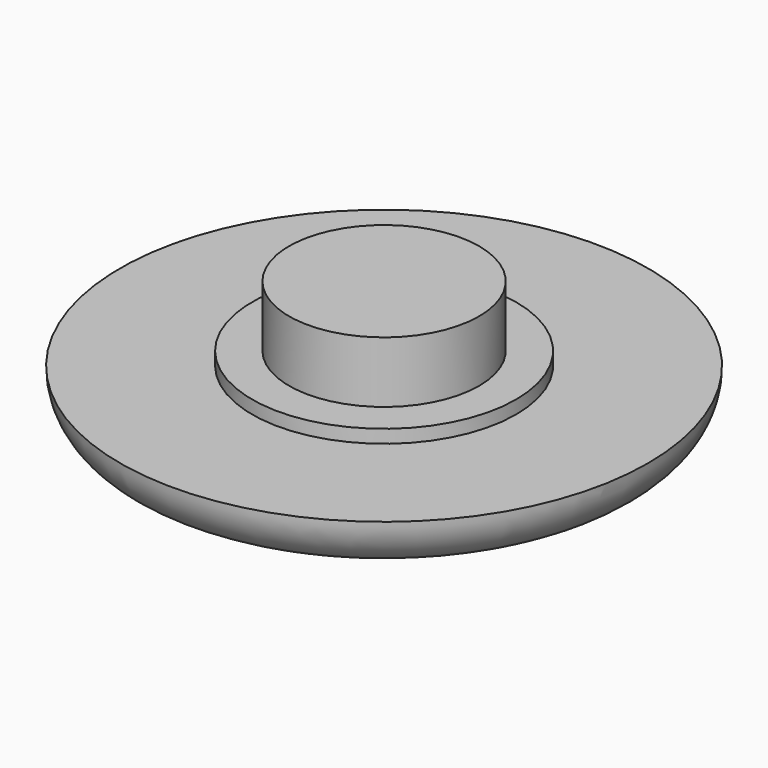
from build123d import *

# Parameters (mm, degrees)
F0_R      = 12.7
F1_DEPTH  = 2.54
F2_R      = 2.53999
F3_R      = 6.35
F4_DEPTH  = 0.635
F5_R      = 4.7625
F6_DEPTH  = 4.7244
F7_R      = 4.7625
F7_R_2    = 4.572
F8_DEPTH  = 4.7244
F9_R      = 4.572
F10_DEPTH = 1.778


# Not quite as in the source:
# - a fillet or chamfer is up to 0.001 mm smaller than in the source, because OpenCascade refuses the exact size


with BuildPart() as f1:
    # F0 (on Top) → F1 (new body)
    with BuildSketch(Plane.XY):
        Circle(F0_R)
    extrude(amount=F1_DEPTH)

    # F2 (radius 2.54 in the source; OpenCascade refuses exactly that, so slightly less here)
    f2_edges = [f1.edges().sort_by_distance(p)[0] for p in [
        (-12.7, 0, 0),
    ]]
    fillet(f2_edges, radius=F2_R)

    # F3 (on face) → F4 (join)
    with BuildSketch(Plane.XY.offset(2.54)):
        Circle(F3_R)
    extrude(amount=F4_DEPTH)

    # F5 (on face) → F6 (join)
    with BuildSketch(Plane.XY.offset(3.175)):
        Circle(F5_R)
    extrude(amount=F6_DEPTH)

    # F7 (on face) → F8 (cut, through all)
    with BuildSketch(Plane.XY.offset(7.8994)):
        Circle(F7_R)
        Circle(F7_R_2, mode=Mode.SUBTRACT)
    extrude(amount=-F8_DEPTH, mode=Mode.SUBTRACT)

    # F9 (on face) → F10 (cut)
    with BuildSketch(Plane.XY.offset(7.8994)):
        Circle(F9_R)
    extrude(amount=-F10_DEPTH, mode=Mode.SUBTRACT)


solid = f1.part
